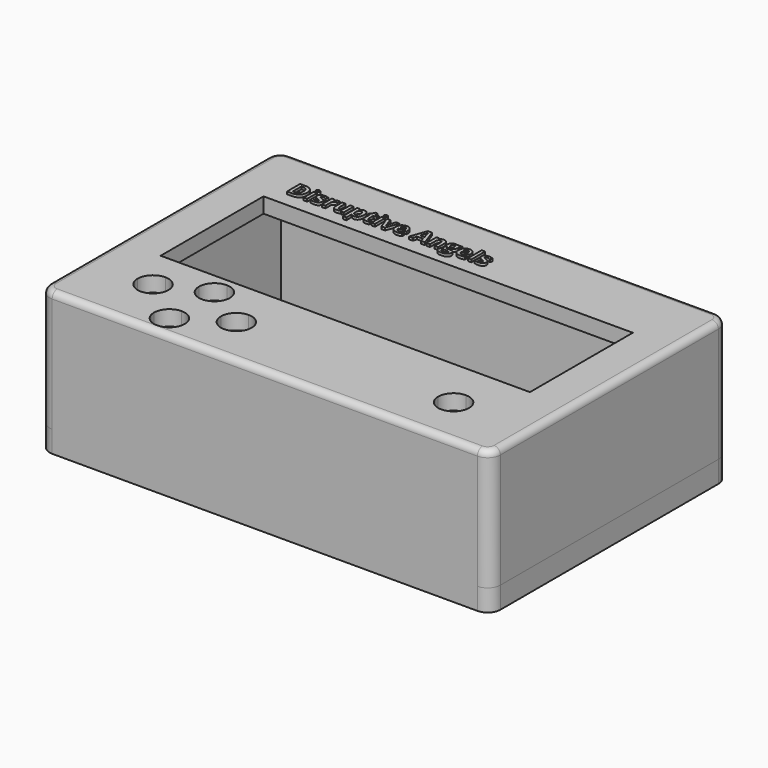
from build123d import *

# Parameters (mm, degrees)
F0_W         = 89.916
F0_H         = 59.436
F0_W_2       = 83.82
F0_H_2       = 53.34
F1_DEPTH     = 3.048
F2_DEPTH     = 17.78
F3_W         = 89.916
F3_H         = 59.436
F3_W_2       = 83.82
F3_H_2       = 53.34
F3_W_3       = 73.66
F3_H_3       = 25.654
F4_DEPTH     = 3.048
F5_TEXT_SIZE = 4.5443108926
F6_DEPTH     = 0.508
F7_DEPTH     = 3.048
F8_DEPTH     = 3.302
F9_DEPTH     = 3.302
F10_R        = 2.54
F11_DEPTH    = 4.318
F12_R        = 1.27


# Not quite as in the source:
# - Text() gives the source's letters only with a copy of the font that has no kerning and outlines rounded to 1/6400 em; it was checked with that copy


with BuildPart() as f1:
    # F0 (on Top) → F1 (new body)
    with BuildSketch(Plane.XY):
        with Locations((-44.958, 29.718)):
            Rectangle(F0_W, F0_H)
        with Locations((-44.958, 29.718)):
            Rectangle(F0_W_2, F0_H_2, mode=Mode.SUBTRACT)
        with Locations((-44.958, 29.718)):
            Rectangle(F0_W_2, F0_H_2)
    extrude(amount=F1_DEPTH)

    # F0 (on Top) → F2 (join)
    with BuildSketch(Plane.XY):
        with Locations((-44.958, 29.718)):
            Rectangle(F0_W, F0_H)
        with Locations((-44.958, 29.718)):
            Rectangle(F0_W_2, F0_H_2, mode=Mode.SUBTRACT)
    extrude(amount=F2_DEPTH)

    # F3 (on face) → F4 (join)
    with BuildSketch(Plane.XY.offset(17.78)):
        with Locations((-44.958, 29.718)):
            Rectangle(F3_W, F3_H)
        with Locations((-44.958, 29.718)):
            Rectangle(F3_W_2, F3_H_2, mode=Mode.SUBTRACT)
        with Locations((-44.958, 29.718)):
            Rectangle(F3_W_2, F3_H_2)
        with Locations((-44.958, 32.893)):
            Rectangle(F3_W_3, F3_H_3, mode=Mode.SUBTRACT)
    extrude(amount=F4_DEPTH)

    # F5 (on face) → F6 (join)
    with BuildSketch(Plane.XY.offset(20.828)):
        with Locations((-79.756, 48.5440961573)):
            Text('Disruptive Angels', F5_TEXT_SIZE, font='Open Sans', font_style=FontStyle.BOLD, text_align=(TextAlign.LEFT, TextAlign.BOTTOM))
    extrude(amount=F6_DEPTH)

    # F5 (on face) → F7 (cut)
    with BuildSketch(Plane.XY.offset(20.828)):
        with BuildLine():
            ThreePointArc((-73.6182862101, 12.0152286757), (-74.5926360434, 14.0382176997), (-76.6828385442, 14.8585198969))
            ThreePointArc((-76.6828385442, 14.8585198969), (-78.8558918493, 13.9584117462), (-79.756, 11.7853584411))
            ThreePointArc((-79.756, 11.7853584411), (-78.8558918493, 9.612305136), (-76.6828385442, 8.7121969853))
            ThreePointArc((-76.6828385442, 8.7121969853), (-74.5926360434, 9.5324991825), (-73.6182862101, 11.5554882065))
            Line((-73.6182862101, 11.5554882065), (-73.6182862101, 12.0152286757))
        make_face()
        with BuildLine():
            ThreePointArc((-64.4742862101, 15.6718), (-65.3744642288, 17.8450219813), (-67.5476862101, 18.7452))
            ThreePointArc((-67.5476862101, 18.7452), (-69.7209081914, 17.8450219813), (-70.6210862101, 15.6718))
            ThreePointArc((-70.6210862101, 15.6718), (-69.7209081914, 13.4985780187), (-67.5476862101, 12.5984))
            ThreePointArc((-67.5476862101, 12.5984), (-65.3744642288, 13.4985780187), (-64.4742862101, 15.6718))
        make_face()
        with BuildLine():
            ThreePointArc((-55.5334862101, 9.9667270999), (-56.4336642288, 12.1399490812), (-58.6068862101, 13.0401270999))
            ThreePointArc((-58.6068862101, 13.0401270999), (-60.7801081914, 12.1399490812), (-61.6802862101, 9.9667270999))
            ThreePointArc((-61.6802862101, 9.9667270999), (-60.7801081914, 7.7935051186), (-58.6068862101, 6.8933270999))
            ThreePointArc((-58.6068862101, 6.8933270999), (-56.4336642288, 7.7935051186), (-55.5334862101, 9.9667270999))
        make_face()
        with BuildLine():
            ThreePointArc((-64.4742862101, 4.445), (-65.3744642288, 6.6182219813), (-67.5476862101, 7.5184))
            ThreePointArc((-67.5476862101, 7.5184), (-69.7209081914, 6.6182219813), (-70.6210862101, 4.445))
            ThreePointArc((-70.6210862101, 4.445), (-69.7209081914, 2.2717780187), (-67.5476862101, 1.3716))
            ThreePointArc((-67.5476862101, 1.3716), (-65.3744642288, 2.2717780187), (-64.4742862101, 4.445))
        make_face()
        with BuildLine():
            ThreePointArc((-12.192, 9.9568), (-13.0921780187, 12.1300219813), (-15.2654, 13.0302))
            ThreePointArc((-15.2654, 13.0302), (-17.4386219813, 12.1300219813), (-18.3388, 9.9568))
            ThreePointArc((-18.3388, 9.9568), (-17.4386219813, 7.7835780187), (-15.2654, 6.8834))
            ThreePointArc((-15.2654, 6.8834), (-13.0921780187, 7.7835780187), (-12.192, 9.9568))
        make_face()
    extrude(amount=-F7_DEPTH, mode=Mode.SUBTRACT)

    # F0 (on Top) → F8 (cut)
    with BuildSketch(Plane.XY):
        with Locations((-44.958, 29.718)):
            Rectangle(F0_W, F0_H)
        with Locations((-44.958, 29.718)):
            Rectangle(F0_W_2, F0_H_2, mode=Mode.SUBTRACT)
        with Locations((-44.958, 29.718)):
            Rectangle(F0_W_2, F0_H_2)
    extrude(amount=F8_DEPTH, mode=Mode.SUBTRACT)

    # F0 (on Top) → F9 (join, symmetric)
    with BuildSketch(Plane.XY):
        with Locations((-44.958, 29.718)):
            Rectangle(F0_W, F0_H)
        with Locations((-44.958, 29.718)):
            Rectangle(F0_W_2, F0_H_2, mode=Mode.SUBTRACT)
    extrude(amount=F9_DEPTH, both=True)

    # F10
    f10_edges = [f1.edges().sort_by_distance(p)[0] for p in [
        (0, 0, 8.763),
        (0, 59.436, 8.763),
        (-89.916, 59.436, 8.763),
        (-89.916, 0, 8.763),
    ]]
    fillet(f10_edges, radius=F10_R)

    # F11 (add): a face of the model
    f11_faces = [f1.faces().sort_by_distance(p)[0] for p in [
        (-44.958, 1.0778462391, -3.302),
    ]]
    extrude(f11_faces, amount=F11_DEPTH)

    # F12
    f12_edges = [f1.edges().sort_by_distance(p)[0] for p in [
        (-44.958, 0, 20.828),
    ]]
    fillet(f12_edges, radius=F12_R)


solid = f1.part
